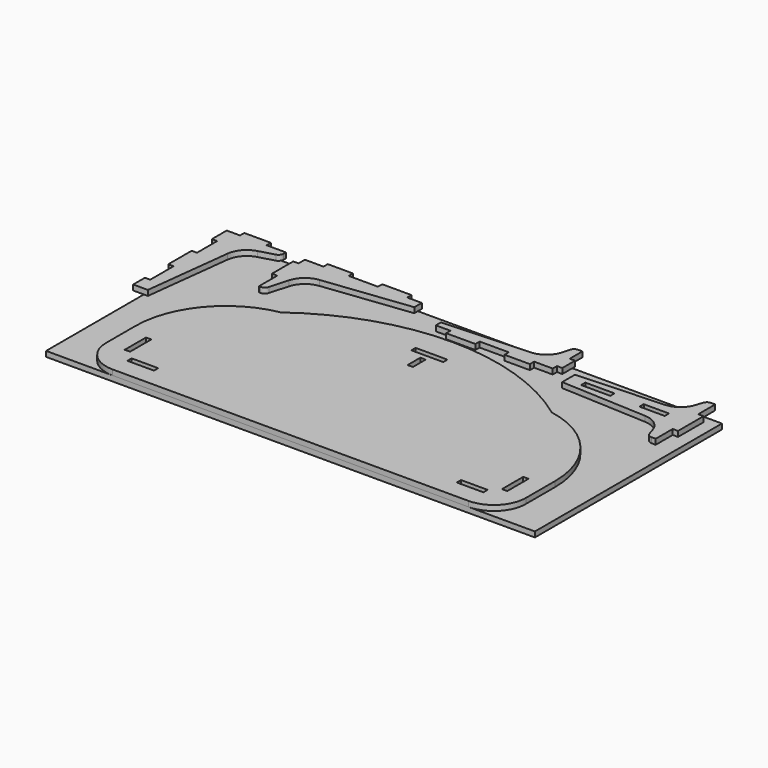
from build123d import *

# Parameters (mm, degrees)
F1_W     = 127
F1_H     = 25.4
F1_W_2   = 25.4
F1_H_2   = 127
F1_H_3   = 76.2
F1_W_3   = 152.4
F2_DEPTH = 25.4
F1_W_4   = 139.7
F1_W_5   = 120.6500786332
F3_W     = 2336.8
F3_H     = 1117.6
F4_DEPTH = 25.4


# Not quite as in the source:
# - a variable given as a bare number and used for a length is read in inches; the dataset says mm whatever the document's units were


with BuildPart() as f2:
    # F1 (on Top) → F2 (new body)
    with BuildSketch(Plane.XY):
        with BuildLine():
            ThreePointArc((647.7, 193.5579180717), (0, 406.4), (-647.7, 193.5579180717))
            ThreePointArc((-647.7, 193.5579180717), (-902.6754821843, 45.6159123042), (-1003.3, -231.4653754076))
            Line((-1003.3, -231.4653754076), (-1003.3, -406.4))
            ThreePointArc((-1003.3, -406.4), (-958.6630734528, -514.1630734528), (-850.9, -558.8))
            Line((-850.9, -558.8), (850.9, -558.8))
            ThreePointArc((850.9, -558.8), (958.6630734528, -514.1630734528), (1003.3, -406.4))
            Line((1003.3, -406.4), (1003.3, -231.4653754076))
            ThreePointArc((1003.3, -231.4653754076), (902.6754821843, 45.6159123042), (647.7, 193.5579180717))
        make_face()
        with Locations((-787.4, -457.2)):
            Rectangle(F1_W, F1_H, mode=Mode.SUBTRACT)
        with Locations((-901.7, -342.9)):
            Rectangle(F1_W_2, F1_H_2, mode=Mode.SUBTRACT)
        with Locations((787.4, -457.2)):
            Rectangle(F1_W, F1_H, mode=Mode.SUBTRACT)
        with Locations((901.7, -342.9)):
            Rectangle(F1_W_2, F1_H_2, mode=Mode.SUBTRACT)
        with Locations((0, 194.9797632933)):
            Rectangle(F1_W_2, F1_H_3, mode=Mode.SUBTRACT)
        with Locations((0, 271.1797632933)):
            Rectangle(F1_W_3, F1_H, mode=Mode.SUBTRACT)
    extrude(amount=F2_DEPTH)


with BuildPart() as f2b:
    # F1 (on Top) → F2, piece 2 (new body)
    with BuildSketch(Plane.XY):
        with BuildLine():
            Line((-1155.7, 584.2), (-1219.2, 584.2))
            Line((-1219.2, 584.2), (-1219.2, 495.3))
            Line((-1219.2, 495.3), (-1193.8, 495.3))
            Line((-1193.8, 495.3), (-1193.8, 374.65))
            Line((-1193.8, 374.65), (-1219.2, 374.65))
            Line((-1219.2, 374.65), (-1219.2, 234.95))
            Line((-1219.2, 234.95), (-1193.8, 234.95))
            Line((-1193.8, 234.95), (-1193.8, 95.25))
            Line((-1193.8, 95.25), (-1219.2, 95.25))
            Line((-1219.2, 95.25), (-1219.2, 25.4))
            Line((-1219.2, 25.4), (-1149.1548928144, 25.4))
            Line((-1149.1548928144, 25.4), (-1100.1678840305, 440.4851537224))
            ThreePointArc((-1100.1678840305, 440.4851537224), (-1076.504269872, 494.5859013387), (-1026.751056115, 526.3896))
            Line((-1026.751056115, 526.3896), (-954.7732654951, 546.6136509902))
            ThreePointArc((-954.7732654951, 546.6136509902), (-941.3995358626, 555.7265307509), (-936.244, 571.0667286567))
            Line((-936.244, 571.0667286567), (-936.244, 584.2))
            Line((-936.244, 584.2), (-1028.7, 584.2))
            Line((-1028.7, 584.2), (-1028.7, 609.6))
            Line((-1028.7, 609.6), (-1155.7, 609.6))
            Line((-1155.7, 609.6), (-1155.7, 584.2))
        make_face()
    extrude(amount=F2_DEPTH)


with BuildPart() as f2c:
    # F1 (on Top) → F2, piece 3 (new body)
    with BuildSketch(Plane.XY):
        with BuildLine():
            Line((-843.9495392799, 307.2166677045), (-835.7073963069, 307.2166677045))
            ThreePointArc((-835.7073963069, 307.2166677045), (-820.3671984011, 312.3722035671), (-811.2543186404, 325.7459331997))
            Line((-811.2543186404, 325.7459331997), (-786.1391392799, 415.1313447704))
            ThreePointArc((-786.1391392799, 415.1313447704), (-754.3354406186, 464.8845585274), (-700.2346930023, 488.5481726859))
            Line((-700.2346930023, 488.5481726859), (-285.1495392799, 537.5351814698))
            Line((-285.1495392799, 537.5351814698), (-285.1495392799, 582.1802886554))
            Line((-285.1495392799, 582.1802886554), (-354.9995392799, 582.1802886554))
            Line((-354.9995392799, 582.1802886554), (-354.9995392799, 607.5802886554))
            Line((-354.9995392799, 607.5802886554), (-494.6995392799, 607.5802886554))
            Line((-494.6995392799, 607.5802886554), (-494.6995392799, 582.1802886554))
            Line((-494.6995392799, 582.1802886554), (-634.3995392799, 582.1802886554))
            Line((-634.3995392799, 582.1802886554), (-634.3995392799, 607.5802886554))
            Line((-634.3995392799, 607.5802886554), (-755.0495392799, 607.5802886554))
            Line((-755.0495392799, 607.5802886554), (-755.0495392799, 582.1802886554))
            Line((-755.0495392799, 582.1802886554), (-843.9495392799, 582.1802886554))
            Line((-843.9495392799, 582.1802886554), (-843.9495392799, 544.0802886554))
            Line((-843.9495392799, 544.0802886554), (-869.3495392799, 544.0802886554))
            Line((-869.3495392799, 544.0802886554), (-869.3495392799, 417.0802886554))
            Line((-869.3495392799, 417.0802886554), (-843.9495392799, 417.0802886554))
            Line((-843.9495392799, 417.0802886554), (-843.9495392799, 307.2166677045))
        make_face()
    extrude(amount=F2_DEPTH)


with BuildPart() as f2d:
    # F1 (on Top) → F2, piece 4 (new body)
    with BuildSketch(Plane.XY):
        with BuildLine():
            Line((524.1474925995, 485.8604307627), (524.1474925995, 447.7604307627))
            Line((524.1474925995, 447.7604307627), (524.1474925995, 409.6604307627))
            Line((524.1474925995, 409.6604307627), (936.7098303317, 390.0960868362))
            ThreePointArc((936.7098303317, 390.0960868362), (993.5014833177, 369.4029146453), (1028.4893234405, 320.1144751514))
            Line((1028.4893234405, 320.1144751514), (1039.1319184416, 287.4843454036))
            ThreePointArc((1039.1319184416, 287.4843454036), (1048.3617125766, 274.8030407518), (1063.2799469204, 269.9604307627))
            Line((1063.2799469204, 269.9604307627), (1082.9474925995, 269.9604307627))
            Line((1082.9474925995, 269.9604307627), (1082.9474925995, 371.5604307627))
            Line((1082.9474925995, 371.5604307627), (1108.3474925995, 371.5604307627))
            Line((1108.3474925995, 371.5604307627), (1108.3474925995, 447.7604307627))
            Line((1108.3474925995, 447.7604307627), (1108.3474925995, 523.9604307627))
            Line((1108.3474925995, 523.9604307627), (1082.9474925995, 523.9604307627))
            Line((1082.9474925995, 523.9604307627), (1082.9474925995, 625.5604307627))
            Line((1082.9474925995, 625.5604307627), (1063.2799469204, 625.5604307627))
            ThreePointArc((1063.2799469204, 625.5604307627), (1048.3617125766, 620.7178207737), (1039.1319184416, 608.0365161219))
            Line((1039.1319184416, 608.0365161219), (1028.4893234405, 575.4063863741))
            ThreePointArc((1028.4893234405, 575.4063863741), (993.5014833177, 526.1179468802), (936.7098303317, 505.4247746893))
            Line((936.7098303317, 505.4247746893), (524.1474925995, 485.8604307627))
        make_face()
        with Locations((663.8474925995, 447.7604307627)):
            Rectangle(F1_W_4, F1_H, mode=Mode.SUBTRACT)
        with Locations((933.7225319161, 447.7604307627)):
            Rectangle(F1_W_5, F1_H, mode=Mode.SUBTRACT)
    extrude(amount=F2_DEPTH)


with BuildPart() as f2e:
    # F1 (on Top) → F2, piece 5 (new body)
    with BuildSketch(Plane.XY):
        with BuildLine():
            ThreePointArc((374.8597252388, 599.0932477678), (340.5029078126, 546.3184624133), (281.6454797612, 523.9271239977))
            Line((281.6454797612, 523.9271239977), (-130.8961626275, 503.931140311))
            Line((-130.8961626275, 503.931140311), (-130.8499912567, 473.1604307627))
            Line((-130.8499912567, 473.1604307628), (-61.0000698899, 473.2652403909))
            Line((-61.0000698899, 473.2652403909), (-61.0000698899, 447.7604307627))
            Line((-61.0000698899, 447.7604307627), (78.6999301101, 447.7604307627))
            Line((78.6999301101, 447.7604307627), (78.6999301101, 473.2652403909))
            Line((78.6999301101, 473.2652403909), (218.3999301101, 473.2652403909))
            Line((218.3999301101, 473.2652403909), (218.3999301101, 447.7604307627))
            Line((218.3999301101, 447.7604307627), (339.0500087433, 447.7604307627))
            Line((339.0500087433, 447.7604307627), (339.0500087433, 473.2652403909))
            Line((339.0500087433, 473.2652403909), (427.9500087433, 473.2652403909))
            Line((427.9500087433, 473.2652403909), (427.9500087433, 498.6652403909))
            Line((427.9500087433, 498.6652403909), (453.3500087433, 498.6652403909))
            Line((453.3500087433, 498.6652403909), (453.3500087433, 574.8652403909))
            Line((453.3500087433, 574.8652403909), (427.9500087433, 574.8652403909))
            Line((427.9500087433, 574.8652403909), (427.9500087433, 651.0652403909))
            Line((427.9500087433, 651.0652403909), (408.2824630643, 651.0652403909))
            ThreePointArc((408.2824630643, 651.0652403909), (392.821845185, 645.8178902115), (383.7492017941, 632.2439250201))
            Line((383.7492017941, 632.2439250201), (374.8597252388, 599.0932477678))
        make_face()
    extrude(amount=F2_DEPTH)


with BuildPart() as f4:
    # F3 (on face) → F4 (new body)
    with BuildSketch(Plane.XY):
        Rectangle(F3_W, F3_H)
    extrude(amount=-F4_DEPTH)


solid = Compound([f2.part, f2b.part, f2c.part, f2d.part, f2e.part, f4.part])
